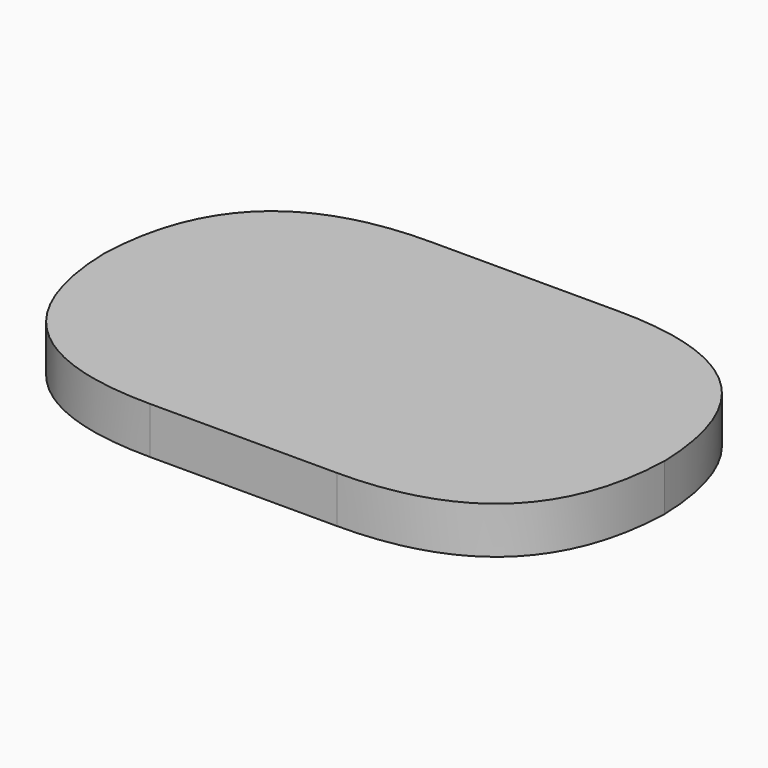
from build123d import *

# Parameters (mm, degrees)
F0_W          = 15.24
F0_H          = 9.525
F1_DEPTH      = 0.635
F1_DEPTH_BACK = 0.635
F2_T1_DEPTH   = 26.67


# Not quite as in the source:
# - a fillet or chamfer that OpenCascade refuses, or shapes differently, is made with other operations: its cross-section is extruded or revolved along the edge and cut away or added


with BuildPart() as f1:
    # F0 (on Top) → F1 (new body, two sides)
    with BuildSketch(Plane.XY) as f1_sk:
        Rectangle(F0_W, F0_H)
    extrude(amount=F1_DEPTH)
    extrude(f1_sk.sketch, amount=-F1_DEPTH_BACK)

    # F2: fillet of radius 5.08 on 4 edges, made by hand

    # F2_s2 → F2_t1 (cut)
    with BuildSketch(Plane.XY.offset(-13.335)):
        with BuildLine():
            add(Edge.make_bspline(
                [(-2.54, -4.7625), (-7.62, -4.7625), (-7.62, 0.3175)],
                knots=[0, 0, 0, 1, 1, 1], degree=2, weights=[1, 1, 1]))
            Line((-7.62, 0.3175), (-7.62, -4.7625))
            Line((-7.62, -4.7625), (-2.54, -4.7625))
        make_face()
        with BuildLine():
            add(Edge.make_bspline(
                [(2.54, -4.7625), (7.62, -4.7625), (7.62, 0.3175)],
                knots=[0, 0, 0, 1, 1, 1], degree=2, weights=[1, 1, 1]))
            Line((7.62, 0.3175), (7.62, -4.7625))
            Line((7.62, -4.7625), (2.54, -4.7625))
        make_face()
        with BuildLine():
            add(Edge.make_bspline(
                [(2.54, 4.7625), (7.62, 4.7625), (7.62, -0.3175)],
                knots=[0, 0, 0, 1, 1, 1], degree=2, weights=[1, 1, 1]))
            Line((7.62, -0.3175), (7.62, 4.7625))
            Line((7.62, 4.7625), (2.54, 4.7625))
        make_face()
        with BuildLine():
            add(Edge.make_bspline(
                [(-2.54, 4.7625), (-7.62, 4.7625), (-7.62, -0.3175)],
                knots=[0, 0, 0, 1, 1, 1], degree=2, weights=[1, 1, 1]))
            Line((-7.62, -0.3175), (-7.62, 4.7625))
            Line((-7.62, 4.7625), (-2.54, 4.7625))
        make_face()
    extrude(amount=F2_T1_DEPTH, mode=Mode.SUBTRACT)


solid = f1.part
